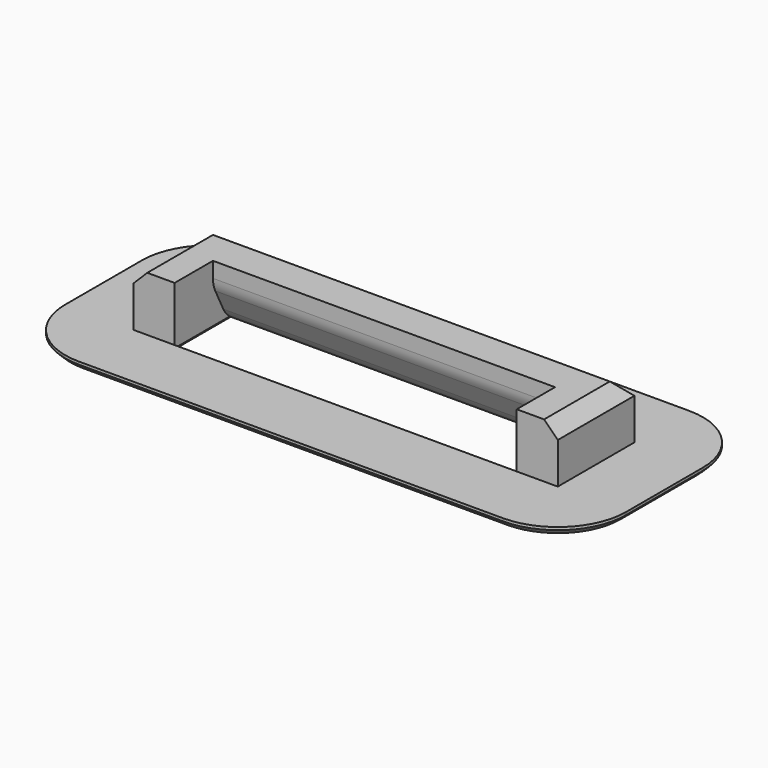
from build123d import *

# Parameters (mm, degrees)
F1_DEPTH = 0.6
F3_DEPTH = 4
F4_SIZE  = 1
F5_SIZE2 = 1.5
F5_SIZE  = 3
F6_R     = 2
F7_W     = 5
F7_H     = 0.6
F8_DEPTH = 25
F9_SIZE  = 0.4


with BuildPart() as f1:
    # F0 (on Top) → F1 (new body)
    with BuildSketch(Plane.XY):
        with BuildLine():
            ThreePointArc((0, 5), (1.4644660941, 1.4644660941), (5, 0))
            Line((5, 0), (8, 0))
            Line((8, 0), (8, 8.5))
            Line((8, 8.5), (33, 8.5))
            Line((33, 8.5), (33, 0))
            Line((33, 0), (36, 0))
            ThreePointArc((36, 0), (39.5355339059, 1.4644660941), (41, 5))
            Line((41, 5), (41, 12))
            ThreePointArc((41, 12), (39.5355339059, 15.5355339059), (36, 17))
            Line((36, 17), (5, 17))
            ThreePointArc((5, 17), (1.4644660941, 15.5355339059), (0, 12))
            Line((0, 12), (0, 5))
        make_face()
    extrude(amount=F1_DEPTH)

    # F2 (on face) → F3 (join)
    with BuildSketch(Plane.XY.offset(0.6)):
        Polygon((36, 12), (5, 12), (5, 5), (8, 5), (8, 8.5), (33, 8.5), (33, 5), (36, 5), align=None)
    extrude(amount=F3_DEPTH)

    # F4
    f4_edges = [f1.edges().sort_by_distance(p)[0] for p in [
        (5, 8.5, 4.6),
        (20.5, 12, 4.6),
        (36, 8.5, 4.6),
    ]]
    chamfer(f4_edges, length=F4_SIZE)

    # F5
    f5_edges = [f1.edges().sort_by_distance(p)[0] for p in [
        (20.5, 8.5, 0),
    ]]
    f5_side = f1.faces().sort_by_distance((20.5, 8.5, 2.3))[0]
    chamfer(f5_edges, length=F5_SIZE, length2=F5_SIZE2, reference=f5_side)

    # F6
    f6_edges = [f1.edges().sort_by_distance(p)[0] for p in [
        (20.5, 10, 0),
        (20.5, 8.5, 3),
    ]]
    fillet(f6_edges, radius=F6_R)

    # F7 (on face) → F8 (join, through all)
    with BuildSketch(Plane.YZ.offset(8)):
        with Locations((2.5, 0.3)):
            Rectangle(F7_W, F7_H)
    extrude(amount=F8_DEPTH)

    # F9
    f9_edges = [f1.edges().sort_by_distance(p)[0] for p in [
        (20.5, 17, 0),
        (20.5, 5, 0),
        (8, 8.118034, 0),
        (41, 8.5, 0),
        (39.535534, 1.464466, 0),
        (20.5, 0, 0),
        (1.464466, 1.464466, 0),
        (0, 8.5, 0),
        (1.464466, 15.535534, 0),
        (39.535534, 15.535534, 0),
        (33, 8.118034, 0),
    ]]
    chamfer(f9_edges, length=F9_SIZE)


solid = f1.part
